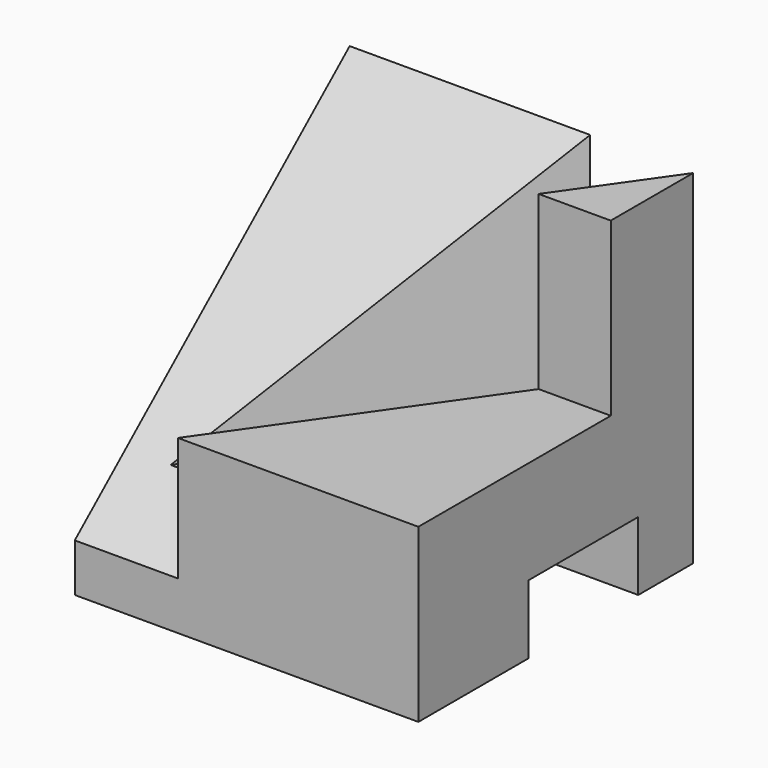
from build123d import *

# Parameters (mm, degrees)
F0_W      = 50
F0_H      = 50
F1_DEPTH  = 50
F3_DEPTH  = 25
F6_DEPTH  = 25
F8_DEPTH  = 25
F9_W      = 20
F9_H      = 10
F11_DEPTH = 30
F13_REACH = 115.9479483752
F14_DEPTH = 35


with BuildPart() as f1:
    # F0 (on Top) → F1 (new body)
    with BuildSketch(Plane.XY):
        with Locations((25, -25)):
            Rectangle(F0_W, F0_H)
    extrude(amount=F1_DEPTH)

    # F2 (on face) → F3 (cut)
    with BuildSketch(Plane.XY.offset(50)):
        Polygon((50, -50), (50, 0), (15, -50), align=None)
    extrude(amount=-F3_DEPTH, mode=Mode.SUBTRACT)

    # F6 (add): a face of the model
    f6_faces = [f1.faces().sort_by_distance(p)[0] for p in [
        (38.3333333333, -33.3333333333, 25),
    ]]
    extrude(f6_faces, amount=F6_DEPTH)

    # F7 (on face) → F8 (cut)
    with BuildSketch(Plane.XY.offset(50)):
        Polygon((15, -50), (50, -50), (50, -15), (39.5, -15), align=None)
    extrude(amount=-F8_DEPTH, mode=Mode.SUBTRACT)

    # F9 (on face) → F11 (cut, through all)
    with BuildSketch(Plane.YZ.offset(50)):
        with Locations((-20, 5)):
            Rectangle(F9_W, F9_H)
    extrude(amount=-F11_DEPTH, mode=Mode.SUBTRACT)

    f13_end = Plane(origin=(27.25, -32.5, 37.5), x_dir=(0.5734623444, 0.8192319205, 0), z_dir=(0.8192319205, -0.5734623444, 0))
    # F12 (on face) → F13 (cut, up to a plane its end follows)
    with BuildSketch(Plane(origin=(0, 0, 0), x_dir=(0, -1, 0), z_dir=(-1, 0, 0))):
        Polygon((50, 50), (0, 50), (50, 7), align=None)
    f13_long = extrude(amount=-F13_REACH, mode=Mode.PRIVATE)
    add(split(f13_long, bisect_by=f13_end, keep=Keep.BOTTOM, mode=Mode.PRIVATE), mode=Mode.SUBTRACT)

    # F4 (on face) → F14 (cut, through all)
    with BuildSketch(Plane.XY.offset(50)):
        Polygon((15, -50), (50, 0), (35, 0), (0, -50), align=None)
    extrude(amount=-F14_DEPTH, mode=Mode.SUBTRACT)


solid = f1.part
